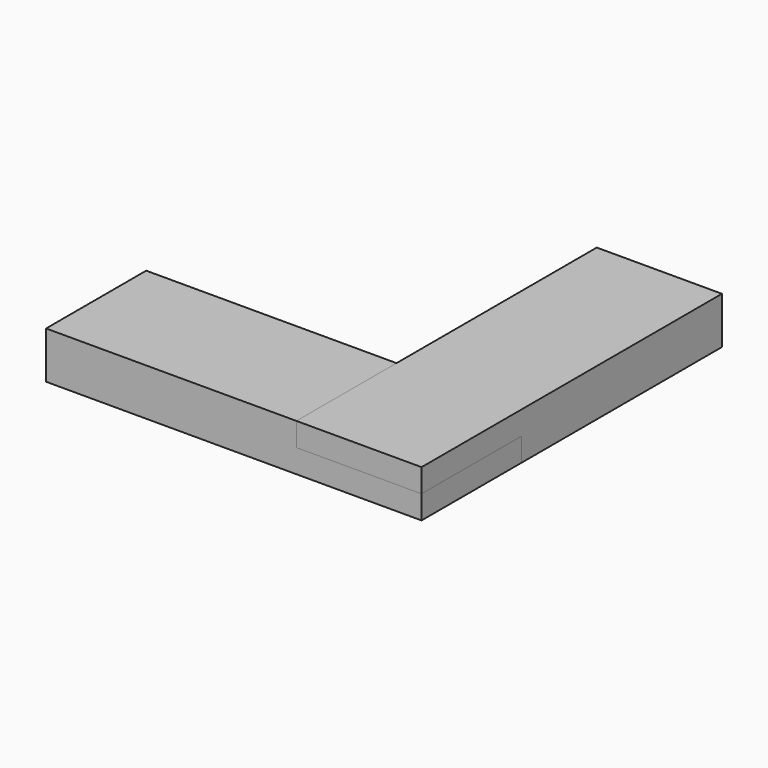
from build123d import *

# Parameters (mm, degrees)
F0_W     = 101.6
F0_H     = 50.8
F1_DEPTH = 9.525
F0_W_2   = 50.8
F2_DEPTH = 9.525
F0_H_2   = 101.6
F3_DEPTH = 9.525
F4_DEPTH = 9.525


with BuildPart() as f1:
    # F0 (on Top) → F1 (new body)
    with BuildSketch(Plane.XY):
        with Locations((-101.6, 25.4)):
            Rectangle(F0_W, F0_H)
    extrude(amount=F1_DEPTH)

    # F0 (on Top) → F2 (join)
    with BuildSketch(Plane.XY):
        with Locations((-25.4, 25.4)):
            Rectangle(F0_W_2, F0_H)
        with Locations((-101.6, 25.4)):
            Rectangle(F0_W, F0_H)
    extrude(amount=-F2_DEPTH)


with BuildPart() as f3:
    # F0 (on Top) → F3 (new body)
    with BuildSketch(Plane.XY):
        with Locations((-25.4, 25.4)):
            Rectangle(F0_W_2, F0_H)
        with Locations((-25.4, 101.6)):
            Rectangle(F0_W_2, F0_H_2)
    extrude(amount=F3_DEPTH)

    # F0 (on Top) → F4 (join)
    with BuildSketch(Plane.XY):
        with Locations((-25.4, 101.6)):
            Rectangle(F0_W_2, F0_H_2)
    extrude(amount=-F4_DEPTH)


solid = Compound([f1.part, f3.part])
